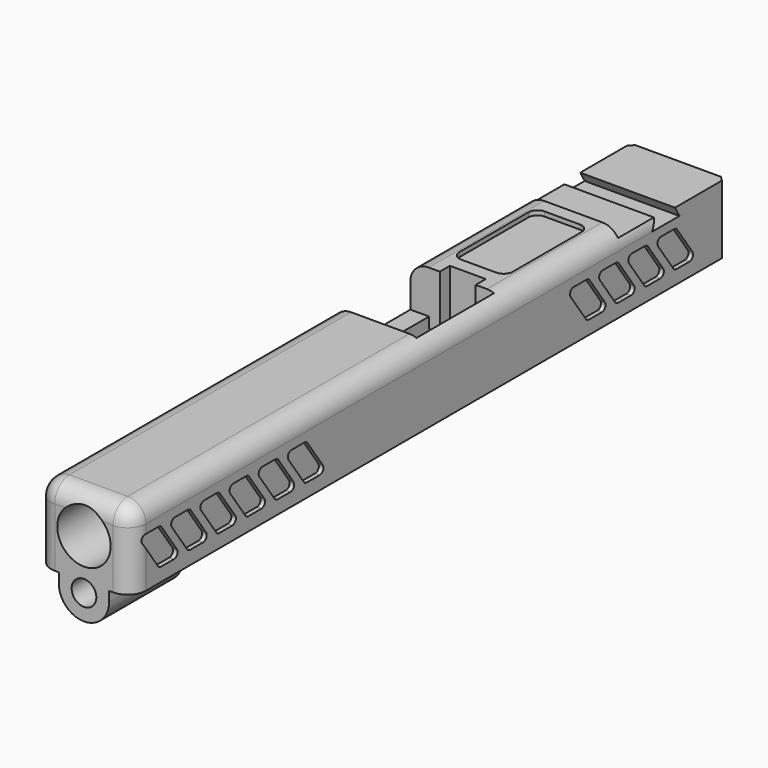
from build123d import *

# Parameters (mm, degrees)
F0_R          = 3.4417
F0_R_2        = 7.4422
F1_DEPTH      = 103.505
F2_W          = 25.654
F2_H          = 9.8319803383
F3_DEPTH      = 57.912
F7_DEPTH      = 25.4
F8_DEPTH      = 18.9992
F10_SIZE      = 2.4892
F6_W          = 2.9972
F6_H          = 2.9972
F6_H_2        = 8.9916
F6_H_3        = 23.5204
F11_DEPTH     = 21.4884
F12_DEPTH     = 6.477
F13_DEPTH     = 1.9812
F15_DEPTH     = 4.064
F16_W         = 36.576
F16_H         = 1.3716
F17_DEPTH     = 44.196
F9_W          = 27.0002
F9_H          = 11.9888
F18_DEPTH     = 1.27
F19_R         = 1.27
F20_W         = 14.8844
F20_H         = 29.0850992904
F21_DEPTH     = 1.27
F22_R         = 2.54
F24_DEPTH     = 25.4
F25_R         = 5.08
F26_SIZE      = 1.27
F27_T1_DEPTH  = 29.1084
F27_T3_DEPTH  = 110.8435007096
F27_T5_DEPTH  = 16.256
F27_T7_DEPTH  = 178.054
F27_T9_DEPTH  = 65.6102992904
F27_S13_W     = 5.08
F27_S13_H     = 5.08
F27_T14_DEPTH = 5.08
F27_S19_W     = 5.08
F27_S19_H     = 5.08
F27_T20_DEPTH = 5.08


# Not quite as in the source:
# - a fillet or chamfer that OpenCascade refuses, or shapes differently, is made with other operations: its cross-section is extruded or revolved along the edge and cut away or added
# - a feature names something its author has since deleted; it is built from what else it names


with BuildPart() as f1:
    # F0 (on Front) → F1 (new body, symmetric)
    with BuildSketch(Plane.XZ):
        with BuildLine():
            Line((13.208, 10.3886), (-13.208, 10.3886))
            Line((-13.208, 10.3886), (-13.208, -11.0998))
            Line((-13.208, -11.0998), (-6.9977, -11.0998))
            Line((-6.9977, -11.0998), (-6.9977, -13.8811))
            ThreePointArc((-6.9977, -13.8811), (0, -20.8788), (6.9977, -13.8811))
            Line((6.9977, -13.8811), (6.9977, -11.0998))
            Line((6.9977, -11.0998), (13.208, -11.0998))
            Line((13.208, -11.0998), (13.208, 10.3886))
        make_face()
        with Locations((0, -13.8811)):
            Circle(F0_R, mode=Mode.SUBTRACT)
        Circle(F0_R_2, mode=Mode.SUBTRACT)
    extrude(amount=F1_DEPTH, both=True)

    # F2 (on face) → F3 (intersect, symmetric)
    with BuildSketch(Plane(origin=(-13.208, 0, 0), x_dir=(0, -1, 0), z_dir=(-1, 0, 0))):
        Polygon((103.505, 10.3886), (-103.505, 10.3886), (-103.505, -11.0998), (77.851, -11.0998), (103.505, -11.0998), align=None)
        with Locations((90.678, -16.0157901691)):
            Rectangle(F2_W, F2_H)
    extrude(amount=F3_DEPTH, both=True, mode=Mode.INTERSECT)

    # F6 (on face) → F7 (cut)
    with BuildSketch(Plane(origin=(0, 0, -11.0998), x_dir=(1, 0, 0), z_dir=(0, 0, -1))):
        Polygon((2.0272319058, 0.2814992904), (-8.001, 0.2814992904), (-8.001, -26.7187007096), (-5.0038, -26.7187007096), (-5.0038, -30.2239007096), (-1.4986, -30.2239007096), (1.4986, -30.2239007096), (2.0272319058, -30.2239007096), align=None)
        Polygon((8.001, 0.2814992904), (2.0272319058, 0.2814992904), (2.0272319058, -30.2239007096), (5.0038, -30.2239007096), (5.0038, -26.7187007096), (8.001, -26.7187007096), align=None)
    extrude(amount=-F7_DEPTH, mode=Mode.SUBTRACT)

    # F6 (on face) → F8 (cut)
    with BuildSketch(Plane(origin=(0, 0, -11.0998), x_dir=(1, 0, 0), z_dir=(0, 0, -1))):
        with BuildLine():
            Line((-10.0076, 67.8434), (-10.0076, 21.2598))
            ThreePointArc((-10.0076, 21.2598), (-9.4927041816, 18.0911054612), (-8.001, 15.2484726291))
            Line((-8.001, 15.2484726291), (-8.001, 0.2814992904))
            Line((-8.001, 0.2814992904), (2.0272319058, 0.2814992904))
            Line((2.0272319058, 0.2814992904), (2.0272319058, 77.6435218645))
            ThreePointArc((2.0272319058, 77.6435218645), (-6.3191902859, 75.6035476719), (-10.0076, 67.8434))
        make_face()
        with BuildLine():
            ThreePointArc((10.0076, 67.8434), (7.7601476719, 74.1625902859), (2.0272319058, 77.6435218645))
            Line((2.0272319058, 77.6435218645), (2.0272319058, 0.2814992904))
            Line((2.0272319058, 0.2814992904), (8.001, 0.2814992904))
            Line((8.001, 0.2814992904), (8.001, 15.2484726291))
            ThreePointArc((8.001, 15.2484726291), (9.4927041816, 18.0911054612), (10.0076, 21.2598))
            Line((10.0076, 21.2598), (10.0076, 67.8434))
        make_face()
    extrude(amount=-F8_DEPTH, mode=Mode.SUBTRACT)

    # F10
    f10_edges = [f1.edges().sort_by_distance(p)[0] for p in [
        (8.001, 13.218601, 10.3886),
    ]]
    chamfer(f10_edges, length=F10_SIZE)

    # F6 (on face) → F11 (join, through all)
    with BuildSketch(Plane(origin=(0, 0, -11.0998), x_dir=(1, 0, 0), z_dir=(0, 0, -1))):
        with Locations((0, -31.7225007096)):
            Rectangle(F6_W, F6_H)
        with Locations((0, -37.7169007096)):
            Rectangle(F6_W, F6_H_2)
        with Locations((0, -53.9729007096)):
            Rectangle(F6_W, F6_H_3)
        Polygon((-5.0038, -26.7187007096), (-8.001, -26.7187007096), (-8.001, -103.505), (2.0272319058, -103.505), (2.0272319058, -30.2239007096), (1.4986, -30.2239007096), (1.4986, -33.2211007096), (1.4986, -42.2127007096), (1.4986, -65.7331007096), (-1.4986, -65.7331007096), (-1.4986, -42.2127007096), (-1.4986, -33.2211007096), (-1.4986, -30.2239007096), (-5.0038, -30.2239007096), align=None)
        Polygon((5.0038, -30.2239007096), (2.0272319058, -30.2239007096), (2.0272319058, -103.505), (8.001, -103.505), (8.001, -26.7187007096), (5.0038, -26.7187007096), align=None)
    extrude(amount=-F11_DEPTH)

    # F6 (on face) → F12 (cut)
    with BuildSketch(Plane(origin=(0, 0, -11.0998), x_dir=(1, 0, 0), z_dir=(0, 0, -1))):
        Polygon((-5.0038, -26.7187007096), (-8.001, -26.7187007096), (-8.001, -103.505), (2.0272319058, -103.505), (2.0272319058, -30.2239007096), (1.4986, -30.2239007096), (1.4986, -33.2211007096), (1.4986, -42.2127007096), (1.4986, -65.7331007096), (-1.4986, -65.7331007096), (-1.4986, -42.2127007096), (-1.4986, -33.2211007096), (-1.4986, -30.2239007096), (-5.0038, -30.2239007096), align=None)
        Polygon((5.0038, -30.2239007096), (2.0272319058, -30.2239007096), (2.0272319058, -103.505), (8.001, -103.505), (8.001, -26.7187007096), (5.0038, -26.7187007096), align=None)
    extrude(amount=-F12_DEPTH, mode=Mode.SUBTRACT)

    # F6 (on face) → F13 (join)
    with BuildSketch(Plane(origin=(0, 0, -11.0998), x_dir=(1, 0, 0), z_dir=(0, 0, -1))):
        with Locations((0, -31.7225007096)):
            Rectangle(F6_W, F6_H)
    extrude(amount=-F13_DEPTH)

    # F14 (on face) → F15 (cut)
    with BuildSketch(Plane(origin=(-1.4986, 0, 0), x_dir=(0, -1, 0), z_dir=(-1, 0, 0))):
        Polygon((-65.7331007096, -11.0998), (-30.2239007096, -11.0998), (-30.2239007096, -9.1186), (-33.2211007096, -9.1186), (-42.2127007096, -7.62), (-65.7331007096, -7.62), align=None)
    extrude(amount=-F15_DEPTH, mode=Mode.SUBTRACT)

    # F16 (on face) → F17 (cut)
    with BuildSketch(Plane(origin=(-13.208, 0, 0), x_dir=(0, -1, 0), z_dir=(-1, 0, 0))):
        with Locations((-85.217, 11.0744)):
            Rectangle(F16_W, F16_H)
        Polygon((-66.929, 10.3886), (-103.505, 10.3886), (-103.505, 7.9502), (-85.8870068321, 7.9502), (-87.4268, 5.2832), (-77.9018, 5.2832), (-79.4415931679, 7.9502), (-66.929, 7.9502), align=None)
    extrude(amount=-F17_DEPTH, mode=Mode.SUBTRACT)

    # F5 (on face) + F9 (on face) → F18 (cut)
    with BuildSketch(Plane(origin=(-13.208, 0, 0), x_dir=(0, -1, 0), z_dir=(-1, 0, 0))):
        Polygon((-86.2308914118, 2.8194), (-93.345, -7.3406), (-85.725, -7.3406), (-78.6108914118, 2.8194), align=None)
        Polygon((-76.0708914118, 2.8194), (-83.185, -7.3406), (-75.565, -7.3406), (-68.4508914118, 2.8194), align=None)
        Polygon((-65.9108914118, 2.8194), (-73.025, -7.3406), (-65.405, -7.3406), (-58.2908914118, 2.8194), align=None)
        Polygon((-55.7508914118, 2.8194), (-62.865, -7.3406), (-55.245, -7.3406), (-48.1308914118, 2.8194), align=None)
        Polygon((52.705, 2.8194), (45.5908914118, -7.3406), (53.2108914118, -7.3406), (60.325, 2.8194), align=None)
        Polygon((62.865, 2.8194), (55.7508914118, -7.3406), (63.3708914118, -7.3406), (70.485, 2.8194), align=None)
        Polygon((73.025, 2.8194), (65.9108914118, -7.3406), (73.5308914118, -7.3406), (80.645, 2.8194), align=None)
        Polygon((83.185, 2.8194), (76.0708914118, -7.3406), (83.6908914118, -7.3406), (90.805, 2.8194), align=None)
        Polygon((42.545, 2.8194), (35.4308914118, -7.3406), (43.0508914118, -7.3406), (50.165, 2.8194), align=None)
        Polygon((93.345, 2.8194), (86.2308914118, -7.3406), (93.8508914118, -7.3406), (100.965, 2.8194), align=None)
    with BuildSketch(Plane.YZ.offset(-8.001)):
        with Locations((13.2186007096, 4.3942)):
            Rectangle(F9_W, F9_H)
    extrude(amount=-F18_DEPTH, dir=(-1, 0, 0), mode=Mode.SUBTRACT)

    # F19
    f19_edges = [f1.edges().sort_by_distance(p)[0] for p in [
        (-12.573, 86.230891, 2.8194),
        (-12.573, 76.070891, 2.8194),
        (-12.573, 65.910891, 2.8194),
        (-12.573, 55.750891, 2.8194),
        (-12.573, 78.610891, 2.8194),
        (-12.573, 68.450891, 2.8194),
        (-12.573, 58.290891, 2.8194),
        (-12.573, 48.130891, 2.8194),
        (-12.573, 55.245, -7.3406),
        (-12.573, 65.405, -7.3406),
        (-12.573, 75.565, -7.3406),
        (-12.573, 85.725, -7.3406),
        (-12.573, 93.345, -7.3406),
        (-12.573, 83.185, -7.3406),
        (-12.573, 73.025, -7.3406),
        (-12.573, 62.865, -7.3406),
        (-12.573, -60.325, 2.8194),
        (-12.573, -70.485, 2.8194),
        (-12.573, -80.645, 2.8194),
        (-12.573, -90.805, 2.8194),
        (-12.573, -83.690891, -7.3406),
        (-12.573, -73.530891, -7.3406),
        (-12.573, -63.370891, -7.3406),
        (-12.573, -53.210891, -7.3406),
        (-12.573, -76.070891, -7.3406),
        (-12.573, -55.750891, -7.3406),
        (-12.573, -45.590891, -7.3406),
        (-12.573, -65.910891, -7.3406),
        (-12.573, -83.185, 2.8194),
        (-12.573, -73.025, 2.8194),
        (-12.573, -62.865, 2.8194),
        (-12.573, -52.705, 2.8194),
        (-12.573, -42.545, 2.8194),
        (-12.573, -100.965, 2.8194),
        (-12.573, -50.165, 2.8194),
        (-12.573, -93.345, 2.8194),
        (-12.573, -86.230891, -7.3406),
        (-12.573, -35.430891, -7.3406),
        (-12.573, -43.050891, -7.3406),
        (-12.573, -93.850891, -7.3406),
    ]]
    fillet(f19_edges, radius=F19_R)

    # F20 (on face) → F21 (cut)
    with BuildSketch(Plane.XY.offset(10.3886)):
        with Locations((0, 48.5764503548)):
            Rectangle(F20_W, F20_H)
    extrude(amount=-F21_DEPTH, mode=Mode.SUBTRACT)

    # F22
    f22_edges = [f1.edges().sort_by_distance(p)[0] for p in [
        (-7.4422, 63.119, 9.7536),
        (7.4422, 34.033901, 9.7536),
        (-7.4422, 34.033901, 9.7536),
        (7.4422, 63.119, 9.7536),
    ]]
    fillet(f22_edges, radius=F22_R)

    # F23: F1 across plane


with BuildPart() as f1_1:
    add(f1.part)
    add(f1.part.mirror(Plane.YZ), mode=Mode.INTERSECT)

    # F9 (on face) → F24 (cut)
    with BuildSketch(Plane.YZ.offset(-8.001)):
        Polygon((26.7187007096, 10.3886), (-0.2814992904, 10.3886), (-0.2814992904, 7.8994), (-0.2814992904, -1.6002), (26.7187007096, -1.6002), align=None)
    extrude(amount=-F24_DEPTH, mode=Mode.SUBTRACT)

    # F25
    f25_edges = [f1_1.edges().sort_by_distance(p)[0] for p in [
        (-10.6045, -0.281499, -1.6002),
    ]]
    fillet(f25_edges, radius=F25_R)

    # F26
    f26_edges = [f1_1.edges().sort_by_distance(p)[0] for p in [
        (-13.208, 103.505, -1.5748),
        (13.208, 103.505, -1.5748),
    ]]
    chamfer(f26_edges, length=F26_SIZE)

    # F27: fillet of radius 5.08 on 6 edges, made by hand

    # F27_s2 → F27_t1 (cut)
    with BuildSketch(Plane.XY.offset(-23.7998)):
        with BuildLine():
            ThreePointArc((-13.208, -98.425), (-11.7201024484, -102.0171024484), (-8.128, -103.505))
            Line((-8.128, -103.505), (-13.208, -103.505))
            Line((-13.208, -103.505), (-13.208, -98.425))
        make_face()
        with BuildLine():
            ThreePointArc((8.128, -103.505), (11.7201024484, -102.0171024484), (13.208, -98.425))
            Line((13.208, -98.425), (13.208, -103.505))
            Line((13.208, -103.505), (8.128, -103.505))
        make_face()
    extrude(amount=F27_T1_DEPTH, mode=Mode.SUBTRACT)

    # F27_s4 → F27_t3 (cut)
    with BuildSketch(Plane.XZ.offset(-12.4185007096)):
        with BuildLine():
            ThreePointArc((-13.208, 5.3086), (-11.7201024484, 8.9007024484), (-8.128, 10.3886))
            Line((-8.128, 10.3886), (-13.208, 10.3886))
            Line((-13.208, 10.3886), (-13.208, 5.3086))
        make_face()
    extrude(amount=F27_T3_DEPTH, mode=Mode.SUBTRACT)

    # F27_s6 → F27_t5 (cut)
    with BuildSketch(Plane.YZ.offset(-8.128)):
        with BuildLine():
            ThreePointArc((-103.505, 5.3086), (-102.0171024484, 8.9007024484), (-98.425, 10.3886))
            Line((-98.425, 10.3886), (-103.505, 10.3886))
            Line((-103.505, 10.3886), (-103.505, 5.3086))
        make_face()
    extrude(amount=F27_T5_DEPTH, mode=Mode.SUBTRACT)

    # F27_s8 → F27_t7 (cut)
    with BuildSketch(Plane.XZ.offset(-79.629)):
        with BuildLine():
            ThreePointArc((8.128, 10.3886), (11.7201024484, 8.9007024484), (13.208, 5.3086))
            Line((13.208, 5.3086), (13.208, 10.3886))
            Line((13.208, 10.3886), (8.128, 10.3886))
        make_face()
    extrude(amount=F27_T7_DEPTH, mode=Mode.SUBTRACT)

    # F27_s10 → F27_t9 (cut)
    with BuildSketch(Plane.XZ.offset(-79.629)):
        with BuildLine():
            ThreePointArc((-13.208, 5.3086), (-11.7201024484, 8.9007024484), (-8.128, 10.3886))
            Line((-8.128, 10.3886), (-13.208, 10.3886))
            Line((-13.208, 10.3886), (-13.208, 5.3086))
        make_face()
    extrude(amount=F27_T9_DEPTH, mode=Mode.SUBTRACT)


with BuildPart() as f27_tool12:
    # F27_s13 → F27_t14 (new body)
    with BuildSketch(Plane.YZ.offset(-8.128)):
        with Locations((-100.965, 7.8486)):
            Rectangle(F27_S13_W, F27_S13_H)
    extrude(amount=-F27_T14_DEPTH)

    # F27_s15 → F27_t16 (revolve, cut)
    with BuildSketch(Plane(origin=(-8.128, -98.425, 5.3086), x_dir=(0, 0.7071067812, -0.7071067812), z_dir=(0, 0.7071067812, 0.7071067812))):
        with BuildLine():
            ThreePointArc((0, -5.08), (5.08, 0), (0, 5.08))
            Line((0, 5.08), (0, -5.08))
        make_face()
    revolve(axis=Axis((-8.128, -98.425, 5.3086), (-1, 0, 0)), mode=Mode.SUBTRACT)


with BuildPart() as f1_2:
    add(f1_1.part)

    # F27_t11: cut F27_tool12
    add(f27_tool12.part, mode=Mode.SUBTRACT)


with BuildPart() as f27_tool18:
    # F27_s19 → F27_t20 (new body)
    with BuildSketch(Plane.YZ.offset(8.128)):
        with Locations((-100.965, 7.8486)):
            Rectangle(F27_S19_W, F27_S19_H)
    extrude(amount=F27_T20_DEPTH)

    # F27_s21 → F27_t22 (revolve, cut)
    with BuildSketch(Plane(origin=(8.128, -98.425, 5.3086), x_dir=(0, 0.7071067812, -0.7071067812), z_dir=(0, -0.7071067812, -0.7071067812))):
        with BuildLine():
            ThreePointArc((0, -5.08), (5.08, 0), (0, 5.08))
            Line((0, 5.08), (0, -5.08))
        make_face()
    revolve(axis=Axis((8.128, -98.425, 5.3086), (1, 0, 0)), mode=Mode.SUBTRACT)


with BuildPart() as f1_3:
    add(f1_2.part)

    # F27_t17: cut F27_tool18
    add(f27_tool18.part, mode=Mode.SUBTRACT)


solid = f1_3.part
